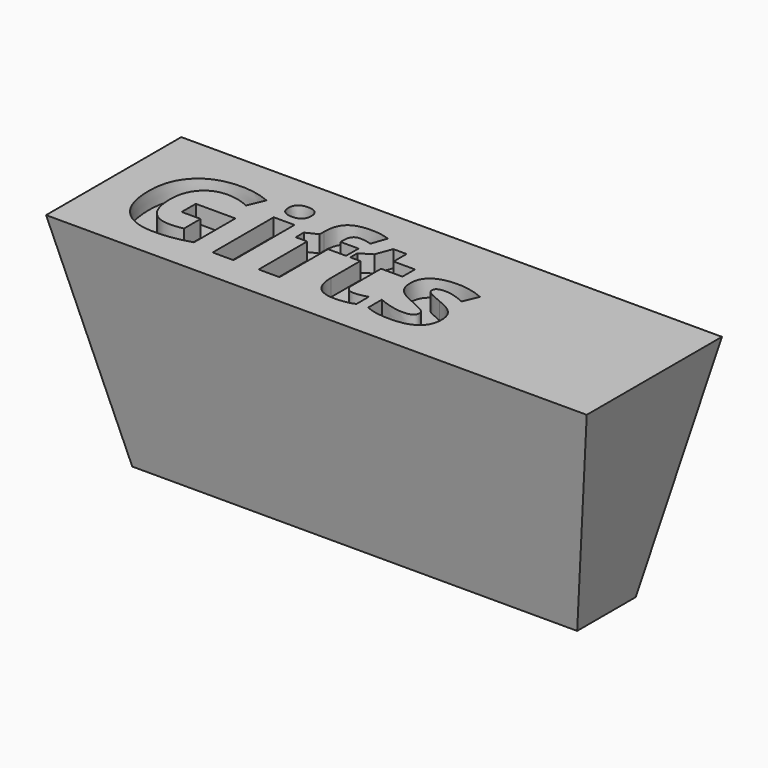
from build123d import *

# Parameters (mm, degrees)
F0_W         = 2438.4
F0_H         = 762
F1_DEPTH     = 1016
F1_TAPER     = 12
F2_TEXT_SIZE = 630.5360752675
F3_DEPTH     = 76.2


# Not quite as in the source:
# - Text() gives the source's letters only with a copy of the font that has no kerning and outlines rounded to 1/6400 em; it was checked with that copy


with BuildPart() as f1:
    # F0 (on Top) → F1 (new body)
    with BuildSketch(Plane.XY):
        Rectangle(F0_W, F0_H)
    extrude(amount=-F1_DEPTH, taper=F1_TAPER)

    # F2 (on face) → F3 (cut)
    with BuildSketch(Plane.XY):
        with Locations((-1088.8220071793, -237.1532917023)):
            Text('Gifts', F2_TEXT_SIZE, font='Open Sans', font_style=FontStyle.BOLD, text_align=(TextAlign.LEFT, TextAlign.BOTTOM))
    extrude(amount=-F3_DEPTH, mode=Mode.SUBTRACT)


solid = f1.part
